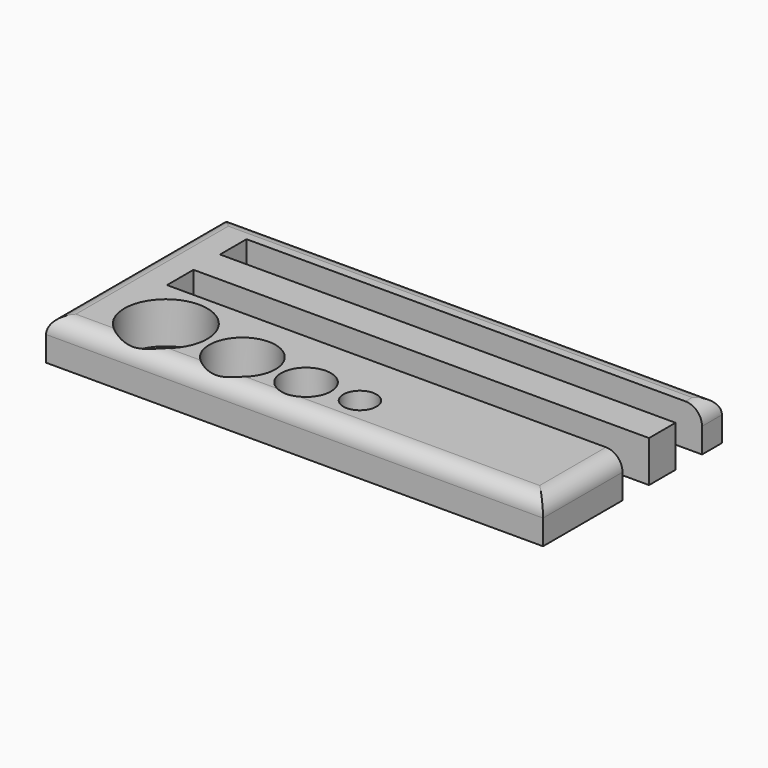
from build123d import *

# Parameters (mm, degrees)
F0_R         = 6.35
F0_R_2       = 5.08
F0_R_3       = 3.81
F0_R_4       = 2.54
F1_DEPTH     = 6.35
F2_T1_DEPTH  = 88.9
F2_T3_DEPTH  = 46.99
F2_T5_DEPTH  = 10.16
F2_T10_DEPTH = 27.94


# Not quite as in the source:
# - a fillet or chamfer that OpenCascade refuses, or shapes differently, is made with other operations: its cross-section is extruded or revolved along the edge and cut away or added


with BuildPart() as f1:
    # F0 (on Top) → F1 (new body)
    with BuildSketch(Plane.XY):
        Polygon((-149.8234506369, 2.128423816), (-73.6234506369, 2.128423816), (-73.6234506369, 17.368423816), (-143.4734506369, 17.368423816), (-143.4734506369, 22.448423816), (-73.6234506369, 22.448423816), (-73.6234506369, 27.528423816), (-143.4734506369, 27.528423816), (-143.4734506369, 32.608423816), (-73.6234506369, 32.608423816), (-73.6234506369, 36.418423816), (-149.8234506369, 36.418423816), align=None)
        with Locations((-137.3288496289, 9.4627772336)):
            Circle(F0_R, mode=Mode.SUBTRACT)
        with Locations((-124.7644872946, 8.4292863984)):
            Circle(F0_R_2, mode=Mode.SUBTRACT)
        with Locations((-114.7297660142, 8.0924675546)):
            Circle(F0_R_3, mode=Mode.SUBTRACT)
        with Locations((-106.7409519207, 8.4292863984)):
            Circle(F0_R_4, mode=Mode.SUBTRACT)
    extrude(amount=F1_DEPTH)

    # F2: fillet of radius 2.54 on 5 edges, made by hand

    # F2_s2 → F2_t1 (cut)
    with BuildSketch(Plane.YZ.offset(-156.1734506369)):
        with BuildLine():
            ThreePointArc((36.418423816, 3.81), (35.6744750402, 5.6060512242), (33.878423816, 6.35))
            Line((33.878423816, 6.35), (36.418423816, 6.35))
            Line((36.418423816, 6.35), (36.418423816, 3.81))
        make_face()
        with BuildLine():
            ThreePointArc((2.128423816, 3.81), (2.8723725918, 5.6060512242), (4.668423816, 6.35))
            Line((4.668423816, 6.35), (2.128423816, 6.35))
            Line((2.128423816, 6.35), (2.128423816, 3.81))
        make_face()
    extrude(amount=F2_T1_DEPTH, mode=Mode.SUBTRACT)

    # F2_s4 → F2_t3 (cut)
    with BuildSketch(Plane.XZ.offset(-42.768423816)):
        with BuildLine():
            ThreePointArc((-149.8234506369, 3.81), (-149.0795018611, 5.6060512242), (-147.2834506369, 6.35))
            Line((-147.2834506369, 6.35), (-149.8234506369, 6.35))
            Line((-149.8234506369, 6.35), (-149.8234506369, 3.81))
        make_face()
    extrude(amount=F2_T3_DEPTH, mode=Mode.SUBTRACT)

    # F2_s6 → F2_t5 (cut)
    with BuildSketch(Plane.XZ.offset(-42.768423816)):
        with BuildLine():
            ThreePointArc((-73.6234506369, 3.81), (-74.3673994126, 5.6060512242), (-76.1634506369, 6.35))
            Line((-76.1634506369, 6.35), (-73.6234506369, 6.35))
            Line((-73.6234506369, 6.35), (-73.6234506369, 3.81))
        make_face()
    extrude(amount=F2_T5_DEPTH, mode=Mode.SUBTRACT)


with BuildPart() as f2_tool8:
    # F2_s9 → F2_t10 (new body)
    with BuildSketch(Plane.XZ.offset(4.221576184)):
        with BuildLine():
            ThreePointArc((-73.6234506369, 3.81), (-74.3673994126, 5.6060512242), (-76.1634506369, 6.35))
            Line((-76.1634506369, 6.35), (-73.6234506369, 6.35))
            Line((-73.6234506369, 6.35), (-73.6234506369, 3.81))
        make_face()
    extrude(amount=-F2_T10_DEPTH)

    split(bisect_by=Plane.XZ.offset(-22.448423816), keep=Keep.TOP)


with BuildPart() as f1_1:
    add(f1.part)

    # F2_t7: cut F2_tool8
    add(f2_tool8.part, mode=Mode.SUBTRACT)


solid = f1_1.part
